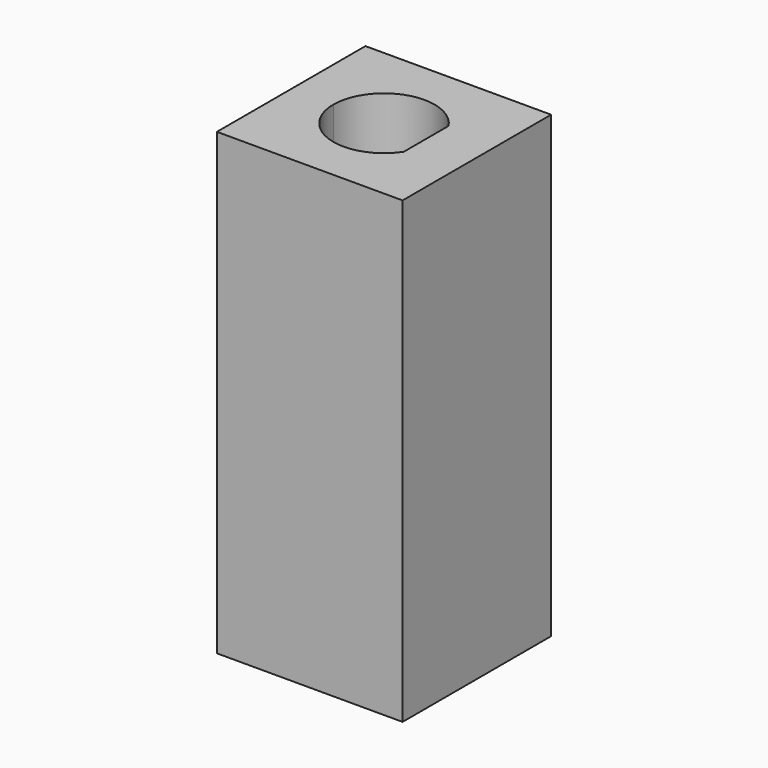
from build123d import *

# Parameters (mm, degrees)
F0_W     = 11
F0_H     = 11
F1_DEPTH = 14.2
F2_W     = 11
F2_H     = 11
F3_DEPTH = 3
F4_W     = 11
F4_H     = 11
F4_W_2   = 3.2
F4_H_2   = 3.2
F5_DEPTH = 10


# Not quite as in the source:
# - a feature names something its author has since deleted; it is built from what else it names


with BuildPart() as f1:
    # F0 (on Top) → F1 (new body)
    with BuildSketch(Plane.XY):
        Rectangle(F0_W, F0_H)
        with BuildLine():
            ThreePointArc((2.5, 1.6583123952), (2.8722813233, 0.8660254038), (3, 0))
            ThreePointArc((3, 0), (2.8722813233, -0.8660254038), (2.5, -1.6583123952))
            ThreePointArc((2.5, -1.6583123952), (-0.8660254038, -2.8722813233), (-3, 0))
            ThreePointArc((-3, 0), (-0.8660254038, 2.8722813233), (2.5, 1.6583123952))
        make_face(mode=Mode.SUBTRACT)
        with BuildLine():
            ThreePointArc((2.5, -1.6583123952), (2.8722813233, -0.8660254038), (3, 0))
            ThreePointArc((3, 0), (2.8722813233, 0.8660254038), (2.5, 1.6583123952))
            Line((2.5, 1.6583123952), (2.5, 0))
            Line((2.5, 0), (2.5, -1.6583123952))
        make_face()
    extrude(amount=F1_DEPTH)

    # F2 (on face) → F3 (join)
    with BuildSketch(Plane(origin=(0, 0, 0), x_dir=(1, 0, 0), z_dir=(0, 0, -1))):
        Rectangle(F2_W, F2_H)
        with BuildLine():
            ThreePointArc((2.5, -1.6583123952), (-3, 0), (2.5, 1.6583123952))
            Line((2.5, 1.6583123952), (2.5, -1.6583123952))
        make_face(mode=Mode.SUBTRACT)
        with BuildLine():
            Line((2.5, -1.6583123952), (2.5, 1.6583123952))
            ThreePointArc((2.5, 1.6583123952), (-3, 0), (2.5, -1.6583123952))
        make_face()
    extrude(amount=F3_DEPTH)

    # F4 (on face) → F5 (join)
    with BuildSketch(Plane(origin=(0, 0, -3), x_dir=(1, 0, 0), z_dir=(0, 0, -1))):
        Rectangle(F4_W, F4_H)
        Rectangle(F4_W_2, F4_H_2, mode=Mode.SUBTRACT)
    extrude(amount=F5_DEPTH)


solid = f1.part
